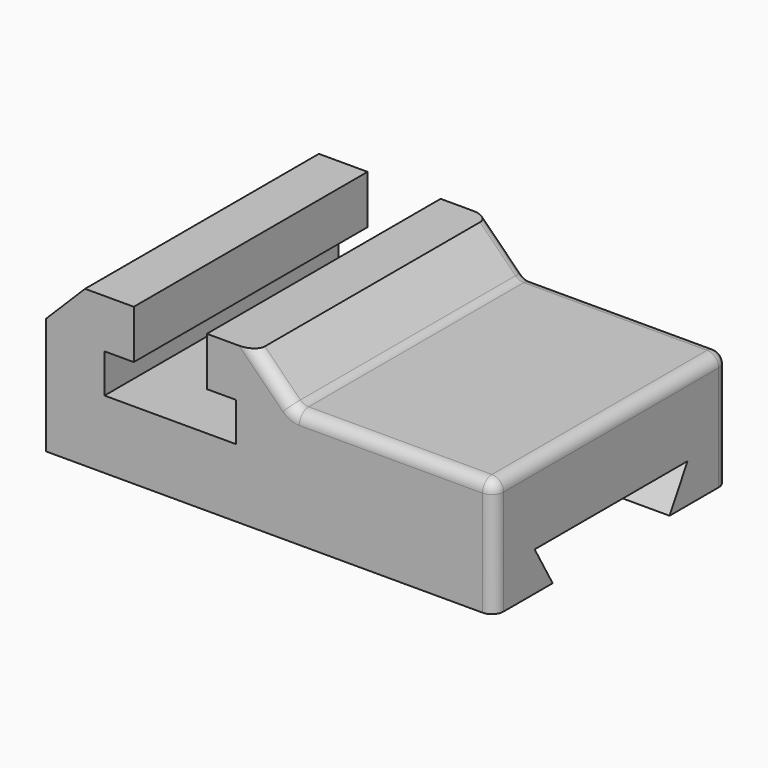
from build123d import *

# Parameters (mm, degrees)
F1_DEPTH = 38.1
F2_R     = 3.048
F4_DEPTH = 116.84


with BuildPart() as f1:
    # F0 (on Front) → F1 (new body, symmetric)
    with BuildSketch(Plane.XZ):
        Polygon((5.08, 10.2046737447), (15.24, 10.2046737447), (5.08, 20.3646737447), align=None)
        Polygon((-49.53, -20.2753262553), (67.31, -20.2753262553), (67.31, 10.2046737447), (15.24, 10.2046737447), (5.08, 10.2046737447), (5.08, 20.3646737447), (-7.62, 20.3646737447), (-7.62, 7.6646737447), (0, 7.6646737447), (0, -2.4953262553), (-34.29, -2.4953262553), (-34.29, 7.6646737447), (-26.67, 7.6646737447), (-26.67, 20.3646737447), (-39.37, 20.3646737447), (-49.53, 10.2046737447), align=None)
    extrude(amount=F1_DEPTH, both=True)

    # F2
    f2_edges = [f1.edges().sort_by_distance(p)[0] for p in [
        (10.16, -38.1, 15.284674),
        (15.24, 0, 10.204674),
        (67.31, -38.1, -5.035326),
        (67.31, 0, 10.204674),
        (41.275, 38.1, 10.204674),
        (67.31, 38.1, -5.035326),
        (10.16, 38.1, 15.284674),
        (41.275, -38.1, 10.204674),
    ]]
    fillet(f2_edges, radius=F2_R)

    # F3 (on face) → F4 (cut)
    with BuildSketch(Plane.YZ.offset(67.31)):
        Polygon((-19.05, -20.2753262553), (0, -20.2753262553), (19.05, -20.2753262553), (19.051521265, -20.2753262553), (24.9174, -10.1153262553), (0, -10.1153262553), (-24.915878735, -10.1153262553), align=None)
    extrude(amount=-F4_DEPTH, mode=Mode.SUBTRACT)


solid = f1.part
